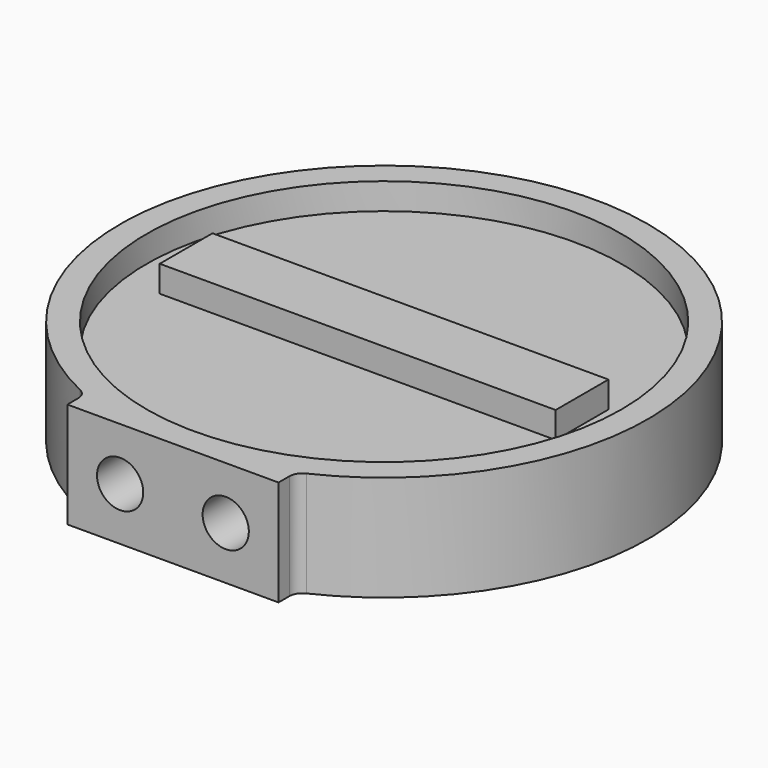
from build123d import *

# Parameters (mm, degrees)
F0_R          = 20
F1_DEPTH      = 8
F2_R          = 18
F2_W          = 30
F2_H          = 5
F3_DEPTH      = 2
F6_END_RADIUS = 18
F5_W          = 16
F5_H          = 8
F6_REACH      = 57.88954382
F7_D          = 3.5
F7_DEPTH      = 8
F7_TIP        = 1.0515060833
F8_R          = 1


with BuildPart() as f1:
    # F0 (on Top) → F1 (new body)
    with BuildSketch(Plane.XY):
        Circle(F0_R)
    extrude(amount=F1_DEPTH)

    # F2 (on face) → F3 (cut)
    with BuildSketch(Plane.XY.offset(8)):
        Circle(F2_R)
        Rectangle(F2_W, F2_H, mode=Mode.SUBTRACT)
    extrude(amount=-F3_DEPTH, mode=Mode.SUBTRACT)

    f6_end = (Plane.XY.offset(7) * Cylinder(F6_END_RADIUS, 230.0419424967, mode=Mode.PRIVATE)).faces().sort_by_distance((-18, 0, 7))[0]
    # F5 (on offset) → F6 (join, up to the whole of a round face its end follows)
    with BuildSketch(Plane.XZ.offset(20)):
        with Locations((0, 4)):
            Rectangle(F5_W, F5_H)
    f6_long = extrude(amount=-F6_REACH, mode=Mode.PRIVATE)
    add(split(f6_long, bisect_by=f6_end, keep=Keep.ALL, mode=Mode.PRIVATE).solids().sort_by_distance((0, -20, 4))[0])

    # F7
    with Locations(Plane.XZ.offset(20)):
        with Locations((4, 4), (-4, 4)):
            Hole(F7_D / 2, depth=F7_DEPTH)
            with Locations((0, 0, -(F7_DEPTH + F7_TIP / 2))):  # 118° drill point
                Cone(0, F7_D / 2, F7_TIP, mode=Mode.SUBTRACT)

    # F8
    f8_edges = [f1.edges().sort_by_distance(p)[0] for p in [
        (8, -18.330303, 4),
        (-8, -18.330303, 4),
    ]]
    fillet(f8_edges, radius=F8_R)


solid = f1.part
